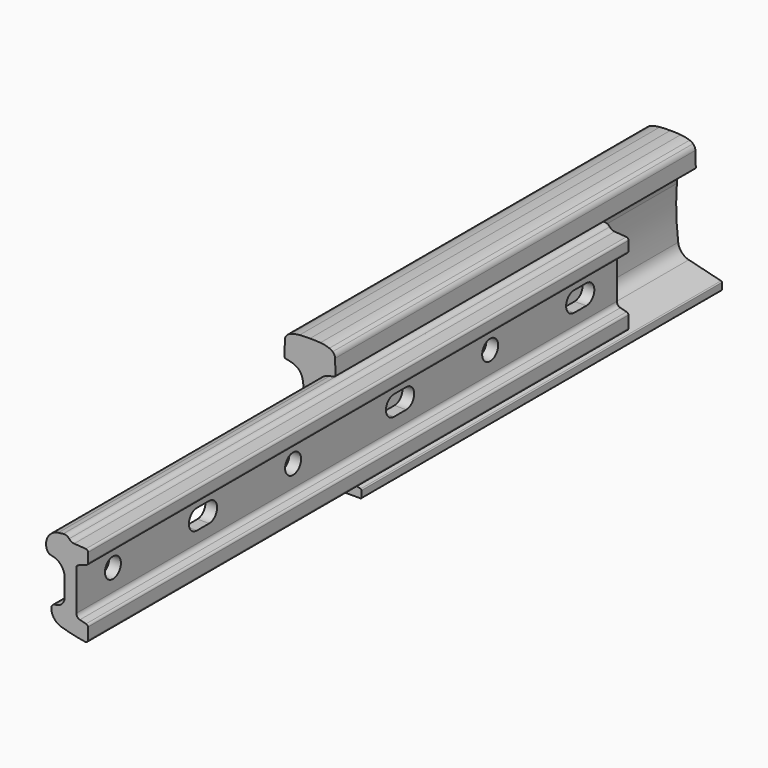
from build123d import *

# Parameters (mm, degrees)
F1_DEPTH  = 609.6
F4_DEPTH  = 609.6
F5_D      = 26.9875
F6_DEPTH  = 609.6
F7_D      = 26.9875
F10_DEPTH = 304.8
F3_R      = 13.49375
F11_DEPTH = 146.051
F12_DEPTH = 457.2
F13_DEPTH = 146.051


with BuildPart() as f1:
    # F0 (on Front) → F1 (new body)
    with BuildSketch(Plane.XZ):
        with BuildLine():
            Line((-68.2625, 0), (0, 0))
            Line((0, 0), (68.2625, 0))
            ThreePointArc((68.2625, 0), (69.3850320151, 0.4649679849), (69.85, 1.5875))
            Line((69.85, 1.5875), (69.85, 9.9184410742))
            ThreePointArc((69.85, 9.9184410742), (69.5134718097, 10.8957976014), (68.6465659448, 11.4587818157))
            Line((68.6465659448, 11.4587818157), (24.9743506964, 22.3479378062))
            ThreePointArc((24.9743506964, 22.3479378062), (15.3287636354, 28.1941789267), (10.6800651686, 38.4706319897))
            ThreePointArc((10.6800651686, 38.4706319897), (8.0613556905, 73.1653941561), (8.8458028883, 107.95))
            ThreePointArc((8.8458028883, 107.95), (9.2700615774, 112.1992308855), (9.9316935792, 116.4180223768))
            ThreePointArc((9.9316935792, 116.4180223768), (14.7844350747, 125.991273848), (24.0421968595, 131.4217517727))
            Line((24.0421968595, 131.4217517727), (33.2061941813, 133.7122565661))
            ThreePointArc((33.2061941813, 133.7122565661), (34.1431824795, 134.329695527), (34.4883874627, 135.3974087192))
            Line((34.4883874627, 135.3974087192), (33.9828374446, 155.6019480071))
            ThreePointArc((33.9828374446, 155.6019480071), (33.0916641168, 159.3928500179), (30.7578125, 162.510263142))
            ThreePointArc((30.7578125, 162.510263142), (28.6026107853, 164.0779738902), (26.19375, 165.2181498143))
            ThreePointArc((26.19375, 165.2181498143), (20.2311975307, 166.9253362084), (14.0890625, 167.7859723667))
            ThreePointArc((14.0890625, 167.7859723667), (7.0487734776, 168.1527062911), (0, 168.275))
            ThreePointArc((0, 168.275), (-7.0487734776, 168.1527062911), (-14.0890625, 167.7859723667))
            ThreePointArc((-14.0890625, 167.7859723667), (-20.2311975307, 166.9253362084), (-26.19375, 165.2181498143))
            ThreePointArc((-26.19375, 165.2181498143), (-28.6026107853, 164.0779738902), (-30.7578125, 162.510263142))
            ThreePointArc((-30.7578125, 162.510263142), (-33.0916641168, 159.3928500179), (-33.9828374446, 155.6019480071))
            Line((-33.9828374446, 155.6019480071), (-34.4883874627, 135.3974087192))
            ThreePointArc((-34.4883874627, 135.3974087192), (-34.1431824795, 134.329695527), (-33.2061941813, 133.7122565661))
            Line((-33.2061941813, 133.7122565661), (-24.0421968595, 131.4217517727))
            ThreePointArc((-24.0421968595, 131.4217517727), (-14.7844350747, 125.991273848), (-9.9316935792, 116.4180223768))
            ThreePointArc((-9.9316935792, 116.4180223768), (-9.2700615774, 112.1992308855), (-8.8458028883, 107.95))
            ThreePointArc((-8.8458028883, 107.95), (-8.0613556905, 73.1653941561), (-10.6800651686, 38.4706319897))
            ThreePointArc((-10.6800651686, 38.4706319897), (-15.3287636354, 28.1941789267), (-24.9743506964, 22.3479378062))
            Line((-24.9743506964, 22.3479378062), (-68.6465659448, 11.4587818157))
            ThreePointArc((-68.6465659448, 11.4587818157), (-69.5134718097, 10.8957976014), (-69.85, 9.9184410742))
            Line((-69.85, 9.9184410742), (-69.85, 1.5875))
            ThreePointArc((-69.85, 1.5875), (-69.3850320151, 0.4649679849), (-68.2625, 0))
        make_face()
    extrude(amount=-F1_DEPTH)


with BuildPart() as f4:
    # F0 (on Front) → F4 (new body)
    with BuildSketch(Plane.XZ):
        with BuildLine():
            Line((-68.2625, 0), (0, 0))
            Line((0, 0), (68.2625, 0))
            ThreePointArc((68.2625, 0), (69.3850320151, 0.4649679849), (69.85, 1.5875))
            Line((69.85, 1.5875), (69.85, 9.9184410742))
            ThreePointArc((69.85, 9.9184410742), (69.5134718097, 10.8957976014), (68.6465659448, 11.4587818157))
            Line((68.6465659448, 11.4587818157), (24.9743506964, 22.3479378062))
            ThreePointArc((24.9743506964, 22.3479378062), (15.3287636354, 28.1941789267), (10.6800651686, 38.4706319897))
            ThreePointArc((10.6800651686, 38.4706319897), (8.0613556905, 73.1653941561), (8.8458028883, 107.95))
            ThreePointArc((8.8458028883, 107.95), (9.2700615774, 112.1992308855), (9.9316935792, 116.4180223768))
            ThreePointArc((9.9316935792, 116.4180223768), (14.7844350747, 125.991273848), (24.0421968595, 131.4217517727))
            Line((24.0421968595, 131.4217517727), (33.2061941813, 133.7122565661))
            ThreePointArc((33.2061941813, 133.7122565661), (34.1431824795, 134.329695527), (34.4883874627, 135.3974087192))
            Line((34.4883874627, 135.3974087192), (33.9828374446, 155.6019480071))
            ThreePointArc((33.9828374446, 155.6019480071), (33.0916641168, 159.3928500179), (30.7578125, 162.510263142))
            ThreePointArc((30.7578125, 162.510263142), (28.6026107853, 164.0779738902), (26.19375, 165.2181498143))
            ThreePointArc((26.19375, 165.2181498143), (20.2311975307, 166.9253362084), (14.0890625, 167.7859723667))
            ThreePointArc((14.0890625, 167.7859723667), (7.0487734776, 168.1527062911), (0, 168.275))
            ThreePointArc((0, 168.275), (-7.0487734776, 168.1527062911), (-14.0890625, 167.7859723667))
            ThreePointArc((-14.0890625, 167.7859723667), (-20.2311975307, 166.9253362084), (-26.19375, 165.2181498143))
            ThreePointArc((-26.19375, 165.2181498143), (-28.6026107853, 164.0779738902), (-30.7578125, 162.510263142))
            ThreePointArc((-30.7578125, 162.510263142), (-33.0916641168, 159.3928500179), (-33.9828374446, 155.6019480071))
            Line((-33.9828374446, 155.6019480071), (-34.4883874627, 135.3974087192))
            ThreePointArc((-34.4883874627, 135.3974087192), (-34.1431824795, 134.329695527), (-33.2061941813, 133.7122565661))
            Line((-33.2061941813, 133.7122565661), (-24.0421968595, 131.4217517727))
            ThreePointArc((-24.0421968595, 131.4217517727), (-14.7844350747, 125.991273848), (-9.9316935792, 116.4180223768))
            ThreePointArc((-9.9316935792, 116.4180223768), (-9.2700615774, 112.1992308855), (-8.8458028883, 107.95))
            ThreePointArc((-8.8458028883, 107.95), (-8.0613556905, 73.1653941561), (-10.6800651686, 38.4706319897))
            ThreePointArc((-10.6800651686, 38.4706319897), (-15.3287636354, 28.1941789267), (-24.9743506964, 22.3479378062))
            Line((-24.9743506964, 22.3479378062), (-68.6465659448, 11.4587818157))
            ThreePointArc((-68.6465659448, 11.4587818157), (-69.5134718097, 10.8957976014), (-69.85, 9.9184410742))
            Line((-69.85, 9.9184410742), (-69.85, 1.5875))
            ThreePointArc((-69.85, 1.5875), (-69.3850320151, 0.4649679849), (-68.2625, 0))
        make_face()
    extrude(amount=-F4_DEPTH)

    # F5 (through all)
    with Locations(Plane.YZ.offset(76.2)):
        with Locations((88.9, 73.025), (241.3, 73.025)):
            Hole(F5_D / 2)


with BuildPart() as f6:
    # F0 (on Front) → F6 (new body)
    with BuildSketch(Plane.XZ):
        with BuildLine():
            Line((-68.2625, 0), (0, 0))
            Line((0, 0), (68.2625, 0))
            ThreePointArc((68.2625, 0), (69.3850320151, 0.4649679849), (69.85, 1.5875))
            Line((69.85, 1.5875), (69.85, 9.9184410742))
            ThreePointArc((69.85, 9.9184410742), (69.5134718097, 10.8957976014), (68.6465659448, 11.4587818157))
            Line((68.6465659448, 11.4587818157), (24.9743506964, 22.3479378062))
            ThreePointArc((24.9743506964, 22.3479378062), (15.3287636354, 28.1941789267), (10.6800651686, 38.4706319897))
            ThreePointArc((10.6800651686, 38.4706319897), (8.0613556905, 73.1653941561), (8.8458028883, 107.95))
            ThreePointArc((8.8458028883, 107.95), (9.2700615774, 112.1992308855), (9.9316935792, 116.4180223768))
            ThreePointArc((9.9316935792, 116.4180223768), (14.7844350747, 125.991273848), (24.0421968595, 131.4217517727))
            Line((24.0421968595, 131.4217517727), (33.2061941813, 133.7122565661))
            ThreePointArc((33.2061941813, 133.7122565661), (34.1431824795, 134.329695527), (34.4883874627, 135.3974087192))
            Line((34.4883874627, 135.3974087192), (33.9828374446, 155.6019480071))
            ThreePointArc((33.9828374446, 155.6019480071), (33.0916641168, 159.3928500179), (30.7578125, 162.510263142))
            ThreePointArc((30.7578125, 162.510263142), (28.6026107853, 164.0779738902), (26.19375, 165.2181498143))
            ThreePointArc((26.19375, 165.2181498143), (20.2311975307, 166.9253362084), (14.0890625, 167.7859723667))
            ThreePointArc((14.0890625, 167.7859723667), (7.0487734776, 168.1527062911), (0, 168.275))
            ThreePointArc((0, 168.275), (-7.0487734776, 168.1527062911), (-14.0890625, 167.7859723667))
            ThreePointArc((-14.0890625, 167.7859723667), (-20.2311975307, 166.9253362084), (-26.19375, 165.2181498143))
            ThreePointArc((-26.19375, 165.2181498143), (-28.6026107853, 164.0779738902), (-30.7578125, 162.510263142))
            ThreePointArc((-30.7578125, 162.510263142), (-33.0916641168, 159.3928500179), (-33.9828374446, 155.6019480071))
            Line((-33.9828374446, 155.6019480071), (-34.4883874627, 135.3974087192))
            ThreePointArc((-34.4883874627, 135.3974087192), (-34.1431824795, 134.329695527), (-33.2061941813, 133.7122565661))
            Line((-33.2061941813, 133.7122565661), (-24.0421968595, 131.4217517727))
            ThreePointArc((-24.0421968595, 131.4217517727), (-14.7844350747, 125.991273848), (-9.9316935792, 116.4180223768))
            ThreePointArc((-9.9316935792, 116.4180223768), (-9.2700615774, 112.1992308855), (-8.8458028883, 107.95))
            ThreePointArc((-8.8458028883, 107.95), (-8.0613556905, 73.1653941561), (-10.6800651686, 38.4706319897))
            ThreePointArc((-10.6800651686, 38.4706319897), (-15.3287636354, 28.1941789267), (-24.9743506964, 22.3479378062))
            Line((-24.9743506964, 22.3479378062), (-68.6465659448, 11.4587818157))
            ThreePointArc((-68.6465659448, 11.4587818157), (-69.5134718097, 10.8957976014), (-69.85, 9.9184410742))
            Line((-69.85, 9.9184410742), (-69.85, 1.5875))
            ThreePointArc((-69.85, 1.5875), (-69.3850320151, 0.4649679849), (-68.2625, 0))
        make_face()
    extrude(amount=-F6_DEPTH)

    # F7 (through all)
    with Locations(Plane.YZ.offset(76.2)):
        with Locations((88.9, 73.025), (241.3, 73.025), (393.7, 73.025)):
            Hole(F7_D / 2)


with BuildPart() as f10:
    # F9 (on offset) → F10 (new body, symmetric)
    with BuildSketch(Plane.XZ.offset(1.5875)):
        with BuildLine():
            ThreePointArc((16.9349182397, 39.0294668641), (20.7165389156, 27.8448012266), (30.3897546784, 21.0752888982))
            ThreePointArc((30.3897546784, 21.0752888982), (46.4639935936, 16.8429835973), (62.8015161128, 13.7804808958))
            ThreePointArc((62.8015161128, 13.7804808958), (65.3450131375, 14.5140229973), (66.4485503232, 16.9201956446))
            Line((66.4485503232, 16.9201956446), (66.4485503232, 32.5290197968))
            ThreePointArc((66.4485503232, 32.5290197968), (65.7758595036, 34.4832648596), (64.0428345653, 35.6094137253))
            Line((64.0428345653, 35.6094137253), (55.6114315158, 37.7150358162))
            ThreePointArc((55.6114315158, 37.7150358162), (52.1453816392, 39.9673335475), (50.8, 43.8758236733))
            Line((50.8, 43.8758236733), (50.8, 98.7437220512))
            ThreePointArc((50.8, 98.7437220512), (51.3758175384, 100.5671461739), (52.8944097836, 101.729178429))
            Line((52.8944097836, 101.729178429), (64.5763656299, 105.9574790967))
            ThreePointArc((64.5763656299, 105.9574790967), (66.0949578751, 107.1195113518), (66.6707754135, 108.9429354746))
            Line((66.6707754135, 108.9429354746), (66.6707754135, 121.6316287782))
            ThreePointArc((66.6707754135, 121.6316287782), (65.8198403638, 123.7948086383), (63.7231551887, 124.7984763334))
            Line((63.7231551887, 124.7984763334), (47.8956258258, 125.9348935451))
            ThreePointArc((47.8956258258, 125.9348935451), (44.1448984259, 127.0147045232), (41.1536063337, 129.5219179956))
            ThreePointArc((41.1536063337, 129.5219179956), (37.5768530258, 132.2191504893), (33.1325614148, 132.781733307))
            Line((33.1325614148, 132.781733307), (26.3438926254, 131.8652780696))
            ThreePointArc((26.3438926254, 131.8652780696), (12.7314351186, 123.0723135598), (10.8139561489, 106.9807474878))
            ThreePointArc((10.8139561489, 106.9807474878), (13.2637980715, 103.4029379457), (17.2387817561, 101.6703239459))
            ThreePointArc((17.2387817561, 101.6703239459), (29.8775568144, 94.9089171003), (34.925, 81.4933077293))
            Line((34.925, 81.4933077293), (34.925, 57.4081940021))
            ThreePointArc((34.925, 57.4081940021), (31.33208824, 48.6191748645), (22.611164628, 44.863996617))
            ThreePointArc((22.611164628, 44.863996617), (18.5728374532, 43.1143757151), (16.9349182397, 39.0294668641))
        make_face()
    extrude(amount=F10_DEPTH, both=True)

    # F3 (on offset) → F11 (cut, through all)
    with BuildSketch(Plane.YZ.offset(76.2)):
        with BuildLine():
            Line((-234.1115368706, 86.51875), (-254.8384631294, 86.51875))
            ThreePointArc((-254.8384631294, 86.51875), (-268.3322131294, 73.025), (-254.8384631294, 59.53125))
            Line((-254.8384631294, 59.53125), (-234.1115368706, 59.53125))
            ThreePointArc((-234.1115368706, 59.53125), (-220.6177868706, 73.025), (-234.1115368706, 86.51875))
        make_face()
        with Locations((-92.075, 73.025)):
            Circle(F3_R)
        with BuildLine():
            Line((99.2634631294, 86.51875), (78.5365368706, 86.51875))
            ThreePointArc((78.5365368706, 86.51875), (65.0427868706, 73.025), (78.5365368706, 59.53125))
            Line((78.5365368706, 59.53125), (99.2634631294, 59.53125))
            ThreePointArc((99.2634631294, 59.53125), (112.7572131294, 73.025), (99.2634631294, 86.51875))
        make_face()
        with Locations((241.3, 73.025)):
            Circle(F3_R)
    extrude(amount=-F11_DEPTH, mode=Mode.SUBTRACT)


with BuildPart() as f12:
    # F9 (on offset) → F12 (new body, symmetric)
    with BuildSketch(Plane.XZ.offset(1.5875)):
        with BuildLine():
            ThreePointArc((16.9349182397, 39.0294668641), (20.7165389156, 27.8448012266), (30.3897546784, 21.0752888982))
            ThreePointArc((30.3897546784, 21.0752888982), (46.4639935936, 16.8429835973), (62.8015161128, 13.7804808958))
            ThreePointArc((62.8015161128, 13.7804808958), (65.3450131375, 14.5140229973), (66.4485503232, 16.9201956446))
            Line((66.4485503232, 16.9201956446), (66.4485503232, 32.5290197968))
            ThreePointArc((66.4485503232, 32.5290197968), (65.7758595036, 34.4832648596), (64.0428345653, 35.6094137253))
            Line((64.0428345653, 35.6094137253), (55.6114315158, 37.7150358162))
            ThreePointArc((55.6114315158, 37.7150358162), (52.1453816392, 39.9673335475), (50.8, 43.8758236733))
            Line((50.8, 43.8758236733), (50.8, 98.7437220512))
            ThreePointArc((50.8, 98.7437220512), (51.3758175384, 100.5671461739), (52.8944097836, 101.729178429))
            Line((52.8944097836, 101.729178429), (64.5763656299, 105.9574790967))
            ThreePointArc((64.5763656299, 105.9574790967), (66.0949578751, 107.1195113518), (66.6707754135, 108.9429354746))
            Line((66.6707754135, 108.9429354746), (66.6707754135, 121.6316287782))
            ThreePointArc((66.6707754135, 121.6316287782), (65.8198403638, 123.7948086383), (63.7231551887, 124.7984763334))
            Line((63.7231551887, 124.7984763334), (47.8956258258, 125.9348935451))
            ThreePointArc((47.8956258258, 125.9348935451), (44.1448984259, 127.0147045232), (41.1536063337, 129.5219179956))
            ThreePointArc((41.1536063337, 129.5219179956), (37.5768530258, 132.2191504893), (33.1325614148, 132.781733307))
            Line((33.1325614148, 132.781733307), (26.3438926254, 131.8652780696))
            ThreePointArc((26.3438926254, 131.8652780696), (12.7314351186, 123.0723135598), (10.8139561489, 106.9807474878))
            ThreePointArc((10.8139561489, 106.9807474878), (13.2637980715, 103.4029379457), (17.2387817561, 101.6703239459))
            ThreePointArc((17.2387817561, 101.6703239459), (29.8775568144, 94.9089171003), (34.925, 81.4933077293))
            Line((34.925, 81.4933077293), (34.925, 57.4081940021))
            ThreePointArc((34.925, 57.4081940021), (31.33208824, 48.6191748645), (22.611164628, 44.863996617))
            ThreePointArc((22.611164628, 44.863996617), (18.5728374532, 43.1143757151), (16.9349182397, 39.0294668641))
        make_face()
    extrude(amount=F12_DEPTH, both=True)

    # F3 (on offset) → F13 (cut, through all)
    with BuildSketch(Plane.YZ.offset(76.2)):
        with Locations((-396.875, 73.025)):
            Circle(F3_R)
        with BuildLine():
            Line((-234.1115368706, 86.51875), (-254.8384631294, 86.51875))
            ThreePointArc((-254.8384631294, 86.51875), (-268.3322131294, 73.025), (-254.8384631294, 59.53125))
            Line((-254.8384631294, 59.53125), (-234.1115368706, 59.53125))
            ThreePointArc((-234.1115368706, 59.53125), (-220.6177868706, 73.025), (-234.1115368706, 86.51875))
        make_face()
        with Locations((-92.075, 73.025)):
            Circle(F3_R)
        with BuildLine():
            Line((99.2634631294, 86.51875), (78.5365368706, 86.51875))
            ThreePointArc((78.5365368706, 86.51875), (65.0427868706, 73.025), (78.5365368706, 59.53125))
            Line((78.5365368706, 59.53125), (99.2634631294, 59.53125))
            ThreePointArc((99.2634631294, 59.53125), (112.7572131294, 73.025), (99.2634631294, 86.51875))
        make_face()
        with Locations((241.3, 73.025)):
            Circle(F3_R)
        with BuildLine():
            Line((404.0634631294, 86.51875), (383.3365368706, 86.51875))
            ThreePointArc((383.3365368706, 86.51875), (369.8427868706, 73.025), (383.3365368706, 59.53125))
            Line((383.3365368706, 59.53125), (404.0634631294, 59.53125))
            ThreePointArc((404.0634631294, 59.53125), (417.5572131294, 73.025), (404.0634631294, 86.51875))
        make_face()
    extrude(amount=-F13_DEPTH, mode=Mode.SUBTRACT)


solid = Compound([f1.part, f4.part, f6.part, f10.part, f12.part])
